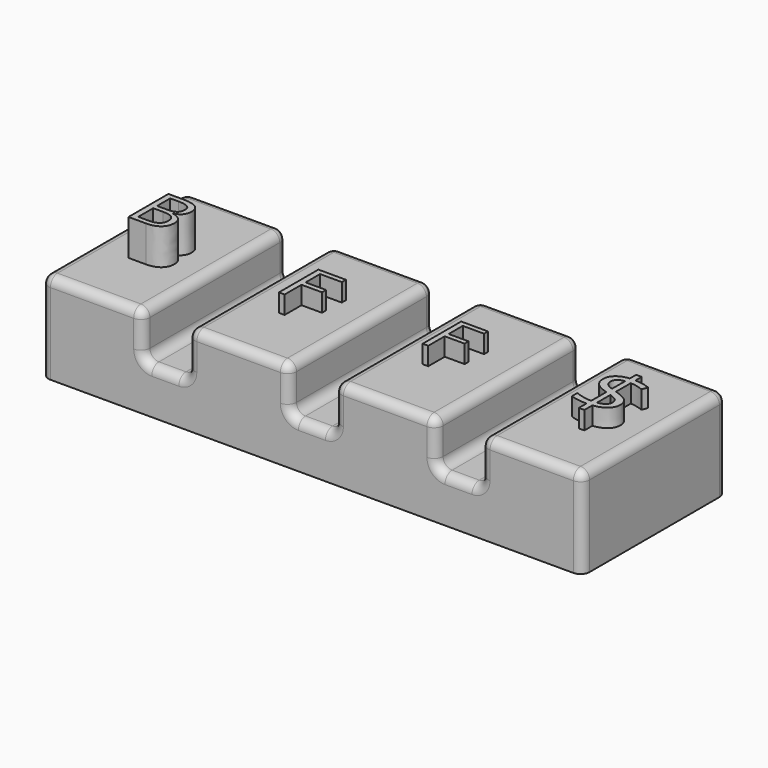
from build123d import *

# Parameters (mm, degrees)
F0_W          = 76.2
F0_H          = 25.4
F1_DEPTH      = 12.7
F2_W          = 6.35
F2_H          = 12.7
F3_DEPTH      = 25.401
F4_R          = 1.27
F5_T          = -2.54
F6_TEXT_SIZE  = 9.8439811457
F7_DEPTH      = 5.08
F8_TEXT_SIZE  = 9.7342621302
F9_DEPTH      = 2.54
F10_TEXT_SIZE = 9.4966051014
F11_DEPTH     = 2.54
F12_TEXT_SIZE = 12.3570285117
F13_DEPTH     = 2.54


# Not quite as in the source:
# - Text() gives the source's letters only with a copy of the font that has no kerning and outlines rounded to 1/6400 em; it was checked with that copy


with BuildPart() as f1:
    # F0 (on Top) → F1 (new body)
    with BuildSketch(Plane.XY):
        Rectangle(F0_W, F0_H)
    extrude(amount=F1_DEPTH)

    # F2 (on face) → F3 (cut, through all)
    with BuildSketch(Plane(origin=(0, 12.7, 0), x_dir=(-1, 0, 0), z_dir=(0, 1, 0))):
        with Locations((0, 12.7)):
            Rectangle(F2_W, F2_H)
        with Locations((20.6502, 12.7)):
            Rectangle(F2_W, F2_H)
        with Locations((-20.6502, 12.7)):
            Rectangle(F2_W, F2_H)
    extrude(amount=-F3_DEPTH, mode=Mode.SUBTRACT)

    # F4
    f4_edges = [f1.edges().sort_by_distance(p)[0] for p in [
        (38.1, 0, 12.7),
        (30.9626, -12.7, 12.7),
        (23.8252, 0, 12.7),
        (30.9626, 12.7, 12.7),
        (17.4752, 0, 12.7),
        (10.3251, -12.7, 12.7),
        (3.175, 0, 12.7),
        (10.3251, 12.7, 12.7),
        (-3.175, 0, 12.7),
        (-10.3251, -12.7, 12.7),
        (-17.4752, 0, 12.7),
        (-10.3251, 12.7, 12.7),
        (20.6502, 12.7, 6.35),
        (17.4752, 0, 6.35),
        (20.6502, -12.7, 6.35),
        (23.8252, 0, 6.35),
        (0, 12.7, 6.35),
        (-3.175, 0, 6.35),
        (0, -12.7, 6.35),
        (3.175, 0, 6.35),
        (-20.6502, 12.7, 6.35),
        (-23.8252, 0, 6.35),
        (-20.6502, -12.7, 6.35),
        (-17.4752, 0, 6.35),
        (-23.8252, 0, 12.7),
        (-30.9626, -12.7, 12.7),
        (-38.1, 0, 12.7),
        (-30.9626, 12.7, 12.7),
        (-38.1, 12.7, 6.35),
        (-38.1, -12.7, 6.35),
        (38.1, 12.7, 6.35),
        (38.1, -12.7, 6.35),
        (-23.8252, 12.7, 9.525),
        (-17.4752, 12.7, 9.525),
        (-3.175, 12.7, 9.525),
        (3.175, 12.7, 9.525),
        (17.4752, 12.7, 9.525),
        (23.8252, 12.7, 9.525),
        (-23.8252, -12.7, 9.525),
        (-17.4752, -12.7, 9.525),
        (-3.175, -12.7, 9.525),
        (3.175, -12.7, 9.525),
        (17.4752, -12.7, 9.525),
        (23.8252, -12.7, 9.525),
    ]]
    fillet(f4_edges, radius=F4_R)

    # F5
    f5_openings = [f1.faces().sort_by_distance(p)[0] for p in [
        (0, 0, 0),
    ]]
    offset(amount=F5_T, openings=f5_openings)

    # F6 (on face) → F7 (join)
    with BuildSketch(Plane.XY.offset(12.7)):
        with Locations((-33.9768547565, -3.722621761)):
            Text('B', F6_TEXT_SIZE, font='Open Sans', text_align=(TextAlign.LEFT, TextAlign.BOTTOM))
    extrude(amount=F7_DEPTH)

    # F8 (on face) → F9 (join)
    with BuildSketch(Plane.XY.offset(12.7)):
        with Locations((-12.8737753257, -3.6042432766)):
            Text('F', F8_TEXT_SIZE, font='Open Sans', text_align=(TextAlign.LEFT, TextAlign.BOTTOM))
    extrude(amount=F9_DEPTH)

    # F10 (on face) → F11 (join)
    with BuildSketch(Plane.XY.offset(12.7)):
        with Locations((7.1360515431, -3.2805840019)):
            Text('F', F10_TEXT_SIZE, font='Open Sans', text_align=(TextAlign.LEFT, TextAlign.BOTTOM))
    extrude(amount=F11_DEPTH)

    # F12 (on face) → F13 (join)
    with BuildSketch(Plane.XY.offset(12.7)):
        with Locations((27.895860374, -3.7748650648)):
            Text('$', F12_TEXT_SIZE, font='Open Sans', text_align=(TextAlign.LEFT, TextAlign.BOTTOM))
    extrude(amount=F13_DEPTH)


solid = f1.part
